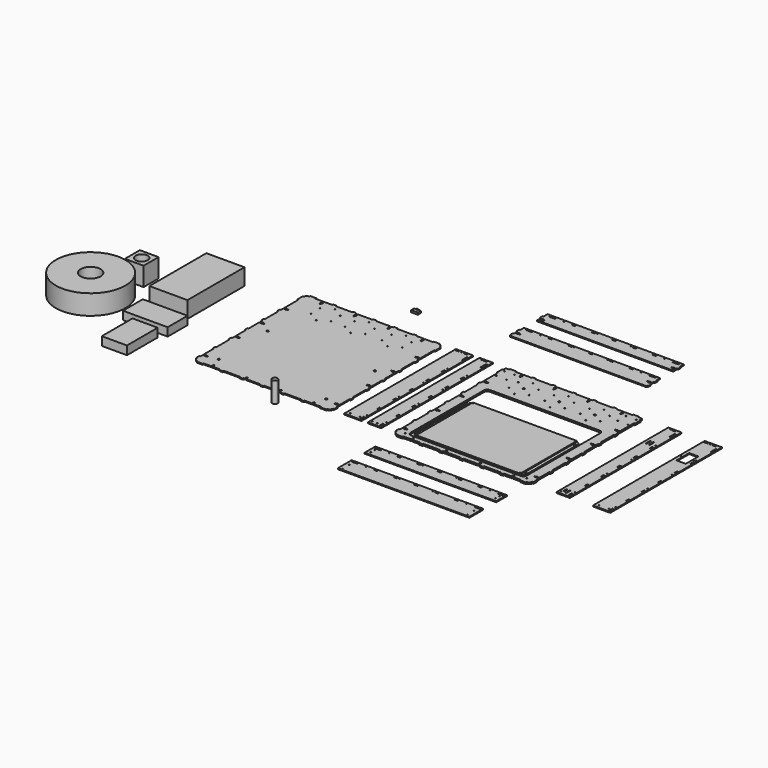
from build123d import *

# Parameters (mm, degrees)
F0_R      = 8
F1_DEPTH  = 62
F2_R      = 1.5
F2_R_2    = 3
F3_DEPTH  = 5
F2_W      = 314
F2_H      = 214
F4_DEPTH  = 2
F2_R_3    = 10
F5_DEPTH  = 3
F2_W_2    = 115
F2_H_2    = 215
F6_DEPTH  = 50
F2_R_4    = 105
F2_R_5    = 30
F7_DEPTH  = 60
F2_W_3    = 135
F2_H_3    = 75
F8_DEPTH  = 25
F2_W_4    = 56.4
F2_H_4    = 56.4
F2_R_6    = 18.5
F9_DEPTH  = 57
F2_W_5    = 76
F2_H_5    = 116
F10_DEPTH = 26
F2_W_6    = 40
F2_H_6    = 408.5
F2_W_7    = 5
F2_H_7    = 13
F2_H_8    = 10
F2_H_9    = 20
F2_H_10   = 12.9999958277
F2_W_8    = 10
F2_H_11   = 3
F11_DEPTH = 3
F2_W_9    = 52
F2_W_10   = 3
F2_W_11   = 28
F2_H_12   = 48
F2_W_12   = 397.0000060797
F2_H_13   = 40
F2_W_13   = 18.5
F2_H_14   = 5
F2_H_15   = 52
F12_DEPTH = 6


# Not quite as in the source:
# - ends of sketch curves that miss each other by under 0.0002 mm in the source are joined
# - a feature names something its author has since deleted; it is built from what else it names


with BuildPart() as f1:
    # F0 (on Top) → F1 (new body)
    with BuildSketch(Plane.XY):
        with Locations((-429.197281599, -257.8284740448)):
            Circle(F0_R)
    extrude(amount=F1_DEPTH)


with BuildPart() as f3:
    # F2 (on Top) → F3 (new body)
    with BuildSketch(Plane.XY):
        with BuildLine():
            Line((102.9999961257, -211.2499983311), (147.2999961257, -211.2499983311))
            Line((147.2999961257, -211.2499983311), (147.2999961257, -208.3499983311))
            Line((147.2999961257, -208.3499983311), (145.7999961257, -208.3499983311))
            Line((145.7999961257, -208.3499983311), (145.7999961257, -205.7499983311))
            Line((145.7999961257, -205.7499983311), (147.2999961257, -205.7499983311))
            Line((147.2999961257, -205.7499983311), (147.2999961257, -202.7499983311))
            Line((147.2999961257, -202.7499983311), (150.6999961257, -202.7499983311))
            Line((150.6999961257, -202.7499983311), (150.6999961257, -205.7499983311))
            Line((150.6999961257, -205.7499983311), (152.1999961257, -205.7499983311))
            Line((152.1999961257, -205.7499983311), (152.1999961257, -208.3499983311))
            Line((152.1999961257, -208.3499983311), (150.6999961257, -208.3499983311))
            Line((150.6999961257, -208.3499983311), (150.6999961257, -211.2499983311))
            Line((150.6999961257, -211.2499983311), (154.9999961257, -211.2499983311))
            Line((154.9999961257, -211.2499983311), (154.9999961257, -214.2499983311))
            Line((154.9999961257, -214.2499983311), (164.9999961257, -214.2499983311))
            Line((164.9999961257, -214.2499983311), (164.9999961257, -211.2499983311))
            Line((164.9999961257, -211.2499983311), (214.9999961257, -211.2499983311))
            Line((214.9999961257, -211.2499983311), (214.9999961257, -214.2499983311))
            Line((214.9999961257, -214.2499983311), (224.9999961257, -214.2499983311))
            Line((224.9999961257, -214.2499983311), (224.9999961257, -211.2499983311))
            Line((224.9999961257, -211.2499983311), (248.2999961257, -211.2499983311))
            Line((248.2999961257, -211.2499983311), (248.2999961257, -208.3499983311))
            Line((248.2999961257, -208.3499983311), (246.7999961257, -208.3499983311))
            Line((246.7999961257, -208.3499983311), (246.7999961257, -205.7499983311))
            Line((246.7999961257, -205.7499983311), (248.2999961257, -205.7499983311))
            Line((248.2999961257, -205.7499983311), (248.2999961257, -202.7499983311))
            Line((248.2999961257, -202.7499983311), (251.6999961257, -202.7499983311))
            Line((251.6999961257, -202.7499983311), (251.6999961257, -205.7499983311))
            Line((251.6999961257, -205.7499983311), (253.1999961257, -205.7499983311))
            Line((253.1999961257, -205.7499983311), (253.1999961257, -208.3499983311))
            Line((253.1999961257, -208.3499983311), (251.6999961257, -208.3499983311))
            Line((251.6999961257, -208.3499983311), (251.6999961257, -211.2499983311))
            Line((251.6999961257, -211.2499983311), (274.9999961257, -211.2499983311))
            Line((274.9999961257, -211.2499983311), (274.9999961257, -214.2499983311))
            Line((274.9999961257, -214.2499983311), (293.4999961257, -214.2499983311))
            Line((293.4999961257, -214.2499983311), (293.4999961257, -211.2499983311))
            ThreePointArc((293.4999961257, -211.2499983311), (300.5710639376, -208.3210661429), (303.4999961257, -201.2499983311))
            Line((303.4999961257, -201.2499983311), (306.4999961257, -201.2499983311))
            Line((306.4999961257, -201.2499983311), (306.4999961257, -188.2500303311))
            Line((306.4999961257, -188.2500303311), (303.4999961257, -188.2500473311))
            Line((303.4999961257, -188.2500473311), (303.4999961257, -179.4499923311))
            Line((303.4999961257, -179.4499923311), (297.0999961257, -179.4499923311))
            Line((297.0999961257, -179.4499923311), (297.0999961257, -180.9499923311))
            Line((297.0999961257, -180.9499923311), (294.4999961257, -180.9499923311))
            Line((294.4999961257, -180.9499923311), (294.4999961257, -179.4499923311))
            Line((294.4999961257, -179.4499923311), (289.4999961257, -179.4499923311))
            Line((289.4999961257, -179.4499923311), (289.4999961257, -176.0499923311))
            Line((289.4999961257, -176.0499923311), (294.4999961257, -176.0499923311))
            Line((294.4999961257, -176.0499923311), (294.4999961257, -174.5499923311))
            Line((294.4999961257, -174.5499923311), (297.0999961257, -174.5499923311))
            Line((297.0999961257, -174.5499923311), (297.0999961257, -176.0499923311))
            Line((297.0999961257, -176.0499923311), (303.4999961257, -176.0499923311))
            Line((303.4999961257, -176.0499923311), (303.4999961257, -138.2500633311))
            Line((303.4999961257, -138.2500633311), (306.4999961257, -138.2500633311))
            Line((306.4999961257, -138.2500633311), (306.4999961257, -128.2500633311))
            Line((306.4999961257, -128.2500633311), (303.4999961257, -128.2500633311))
            Line((303.4999961257, -128.2500633311), (303.4999961257, -78.2500633311))
            Line((303.4999961257, -78.2500633311), (306.4999961257, -78.2500633311))
            Line((306.4999961257, -78.2500633311), (306.4999961257, -68.2500633311))
            Line((306.4999961257, -68.2500633311), (303.4999961257, -68.2500633311))
            Line((303.4999961257, -68.2500633311), (303.4999961257, -58.4499923311))
            Line((303.4999961257, -58.4499923311), (297.0999961257, -58.4499923311))
            Line((297.0999961257, -58.4499923311), (297.0999961257, -59.9499923311))
            Line((297.0999961257, -59.9499923311), (294.4999961257, -59.9499923311))
            Line((294.4999961257, -59.9499923311), (294.4999961257, -58.4499923311))
            Line((294.4999961257, -58.4499923311), (289.4999961257, -58.4499923311))
            Line((289.4999961257, -58.4499923311), (289.4999961257, -55.0499923311))
            Line((289.4999961257, -55.0499923311), (294.4999961257, -55.0499923311))
            Line((294.4999961257, -55.0499923311), (294.4999961257, -53.5499923311))
            Line((294.4999961257, -53.5499923311), (297.0999961257, -53.5499923311))
            Line((297.0999961257, -53.5499923311), (297.0999961257, -55.0499923311))
            Line((297.0999961257, -55.0499923311), (303.4999961257, -55.0499923311))
            Line((303.4999961257, -55.0499923311), (303.4999961257, -16.2500633311))
            Line((303.4999961257, -16.2500633311), (306.4999961257, -16.2500633311))
            Line((306.4999961257, -16.2500633311), (306.4999961257, -6.2500633311))
            Line((306.4999961257, -6.2500633311), (303.4999961257, -6.2500633311))
            Line((303.4999961257, -6.2500633311), (303.4999961257, 33.5500076689))
            Line((303.4999961257, 33.5500076689), (297.0999961257, 33.5500076689))
            Line((297.0999961257, 33.5500076689), (297.0999961257, 32.0500076689))
            Line((297.0999961257, 32.0500076689), (294.4999961257, 32.0500076689))
            Line((294.4999961257, 32.0500076689), (294.4999961257, 33.5500076689))
            Line((294.4999961257, 33.5500076689), (289.4999961257, 33.5500076689))
            Line((289.4999961257, 33.5500076689), (289.4999961257, 36.9500076689))
            Line((289.4999961257, 36.9500076689), (294.4999961257, 36.9500076689))
            Line((294.4999961257, 36.9500076689), (294.4999961257, 38.4500076689))
            Line((294.4999961257, 38.4500076689), (297.0999961257, 38.4500076689))
            Line((297.0999961257, 38.4500076689), (297.0999961257, 36.9500076689))
            Line((297.0999961257, 36.9500076689), (303.4999961257, 36.9500076689))
            Line((303.4999961257, 36.9500076689), (303.4999961257, 45.7499366689))
            Line((303.4999961257, 45.7499366689), (306.4999961257, 45.7499366689))
            Line((306.4999961257, 45.7499366689), (306.4999961257, 55.7499366689))
            Line((306.4999961257, 55.7499366689), (303.4999961257, 55.7499366689))
            Line((303.4999961257, 55.7499366689), (303.4999961257, 105.7499366689))
            Line((303.4999961257, 105.7499366689), (306.4999961257, 105.7499366689))
            Line((306.4999961257, 105.7499366689), (306.4999961257, 115.7499366689))
            Line((306.4999961257, 115.7499366689), (303.4999961257, 115.7499366689))
            Line((303.4999961257, 115.7499366689), (303.4999961257, 124.5500076689))
            Line((303.4999961257, 124.5500076689), (297.0999961257, 124.5500076689))
            Line((297.0999961257, 124.5500076689), (297.0999961257, 123.0500076689))
            Line((297.0999961257, 123.0500076689), (294.4999961257, 123.0500076689))
            Line((294.4999961257, 123.0500076689), (294.4999961257, 124.5500076689))
            Line((294.4999961257, 124.5500076689), (289.4999961257, 124.5500076689))
            Line((289.4999961257, 124.5500076689), (289.4999961257, 127.9500076689))
            Line((289.4999961257, 127.9500076689), (294.4999961257, 127.9500076689))
            Line((294.4999961257, 127.9500076689), (294.4999961257, 129.4500076689))
            Line((294.4999961257, 129.4500076689), (297.0999961257, 129.4500076689))
            Line((297.0999961257, 129.4500076689), (297.0999961257, 127.9500076689))
            Line((297.0999961257, 127.9500076689), (303.4999961257, 127.9500076689))
            Line((303.4999961257, 127.9500076689), (303.4999961257, 181.2500016689))
            Line((303.4999961257, 181.2500016689), (306.4999961257, 181.2500016689))
            Line((306.4999961257, 181.2500016689), (306.4999961257, 201.2500016689))
            Line((306.4999961257, 201.2500016689), (303.4999961257, 201.2500016689))
            Line((303.4999961257, 201.2500016689), (303.4999961257, 211.2500016689))
            Line((303.4999961257, 211.2500016689), (293.4999961257, 211.2500016689))
            Line((293.4999961257, 211.2500016689), (293.4999961257, 214.2500016689))
            Line((293.4999961257, 214.2500016689), (274.9999961257, 214.25))
            Line((274.9999961257, 214.25), (274.9999961257, 211.2500016689))
            Line((274.9999961257, 211.2500016689), (251.6999981257, 211.2500016689))
            Line((251.6999981257, 211.2500016689), (251.6999981257, 204.8500016689))
            Line((251.6999981257, 204.8500016689), (253.1999981257, 204.8500016689))
            Line((253.1999981257, 204.8500016689), (253.1999981257, 202.2500016689))
            Line((253.1999981257, 202.2500016689), (251.6999981257, 202.2500016689))
            Line((251.6999981257, 202.2500016689), (251.6999981257, 197.2500016689))
            Line((251.6999981257, 197.2500016689), (248.2999981257, 197.2500016689))
            Line((248.2999981257, 197.2500016689), (248.2999981257, 202.2500016689))
            Line((248.2999981257, 202.2500016689), (246.7999981257, 202.2500016689))
            Line((246.7999981257, 202.2500016689), (246.7999981257, 204.8500016689))
            Line((246.7999981257, 204.8500016689), (248.2999981257, 204.8500016689))
            Line((248.2999981257, 204.8500016689), (248.2999981257, 211.2500016689))
            Line((248.2999981257, 211.2500016689), (224.9999961257, 211.2500016689))
            Line((224.9999961257, 211.2500016689), (224.9999961257, 214.2500016689))
            Line((224.9999961257, 214.2500016689), (214.9999961257, 214.2500016689))
            Line((214.9999961257, 214.2500016689), (214.9999961257, 211.2500016689))
            Line((214.9999961257, 211.2500016689), (164.9999961257, 211.2500016689))
            Line((164.9999961257, 211.2500016689), (164.9999961257, 214.2500016689))
            Line((164.9999961257, 214.2500016689), (154.9999961257, 214.2500016689))
            Line((154.9999961257, 214.2500016689), (154.9999961257, 211.2500016689))
            Line((154.9999961257, 211.2500016689), (150.6999981257, 211.2500016689))
            Line((150.6999981257, 211.2500016689), (150.6999981257, 204.8500016689))
            Line((150.6999981257, 204.8500016689), (152.1999981257, 204.8500016689))
            Line((152.1999981257, 204.8500016689), (152.1999981257, 202.2500016689))
            Line((152.1999981257, 202.2500016689), (150.6999981257, 202.2500016689))
            Line((150.6999981257, 202.2500016689), (150.6999981257, 197.2500016689))
            Line((150.6999981257, 197.2500016689), (147.2999981257, 197.2500016689))
            Line((147.2999981257, 197.2500016689), (147.2999981257, 202.2500016689))
            Line((147.2999981257, 202.2500016689), (145.7999981257, 202.2500016689))
            Line((145.7999981257, 202.2500016689), (145.7999981257, 204.8500016689))
            Line((145.7999981257, 204.8500016689), (147.2999981257, 204.8500016689))
            Line((147.2999981257, 204.8500016689), (147.2999981257, 211.2500016689))
            Line((147.2999981257, 211.2500016689), (102.9999961257, 211.2500016689))
            Line((102.9999961257, 211.2500016689), (102.9999961257, 214.2500016689))
            Line((102.9999961257, 214.2500016689), (92.9999961257, 214.2500016689))
            Line((92.9999961257, 214.2500016689), (92.9999961257, 211.2500016689))
            Line((92.9999961257, 211.2500016689), (48.6999981257, 211.2500016689))
            Line((48.6999981257, 211.2500016689), (48.6999981257, 204.8500016689))
            Line((48.6999981257, 204.8500016689), (50.1999981257, 204.8500016689))
            Line((50.1999981257, 204.8500016689), (50.1999981257, 202.2500016689))
            Line((50.1999981257, 202.2500016689), (48.6999981257, 202.2500016689))
            Line((48.6999981257, 202.2500016689), (48.6999981257, 197.2500016689))
            Line((48.6999981257, 197.2500016689), (45.2999981257, 197.2500016689))
            Line((45.2999981257, 197.2500016689), (45.2999981257, 202.2500016689))
            Line((45.2999981257, 202.2500016689), (43.7999981257, 202.2500016689))
            Line((43.7999981257, 202.2500016689), (43.7999981257, 204.8500016689))
            Line((43.7999981257, 204.8500016689), (45.2999981257, 204.8500016689))
            Line((45.2999981257, 204.8500016689), (45.2999981257, 211.2500016689))
            Line((45.2999981257, 211.2500016689), (40.9999961257, 211.2500016689))
            Line((40.9999961257, 211.2500016689), (40.9999961257, 214.2500016689))
            Line((40.9999961257, 214.2500016689), (30.9999961257, 214.2500016689))
            Line((30.9999961257, 214.2500016689), (30.9999961257, 211.2500016689))
            Line((30.9999961257, 211.2500016689), (-19.0000038743, 211.2500016689))
            Line((-19.0000038743, 211.2500016689), (-19.0000038743, 214.2500016689))
            Line((-19.0000038743, 214.2500016689), (-29.0000038743, 214.2500016689))
            Line((-29.0000038743, 214.2500016689), (-29.0000038743, 211.2500016689))
            Line((-29.0000038743, 211.2500016689), (-52.3000018743, 211.2500016689))
            Line((-52.3000018743, 211.2500016689), (-52.3000018743, 204.8500016689))
            Line((-52.3000018743, 204.8500016689), (-50.8000018743, 204.8500016689))
            Line((-50.8000018743, 204.8500016689), (-50.8000018743, 202.2500016689))
            Line((-50.8000018743, 202.2500016689), (-52.3000018743, 202.2500016689))
            Line((-52.3000018743, 202.2500016689), (-52.3000018743, 197.2500016689))
            Line((-52.3000018743, 197.2500016689), (-55.7000018743, 197.2500016689))
            Line((-55.7000018743, 197.2500016689), (-55.7000018743, 202.2500016689))
            Line((-55.7000018743, 202.2500016689), (-57.2000018743, 202.2500016689))
            Line((-57.2000018743, 202.2500016689), (-57.2000018743, 204.8500016689))
            Line((-57.2000018743, 204.8500016689), (-55.7000018743, 204.8500016689))
            Line((-55.7000018743, 204.8500016689), (-55.7000018743, 211.2500016689))
            Line((-55.7000018743, 211.2500016689), (-79.0000038743, 211.2500016689))
            Line((-79.0000038743, 211.2500016689), (-79.0000038743, 214.2500016689))
            Line((-79.0000038743, 214.2500016689), (-97.5000038743, 214.2500016689))
            Line((-97.5000038743, 214.2500016689), (-97.5000038743, 211.2500016689))
            Line((-97.5000038743, 211.2500016689), (-107.5000038743, 211.2500016689))
            Line((-107.5000038743, 211.2500016689), (-107.5000038743, 201.2500016689))
            Line((-107.5000038743, 201.2500016689), (-110.5000038743, 201.2500016689))
            Line((-110.5000038743, 201.2500016689), (-110.5000038743, 181.2500016689))
            Line((-110.5000038743, 181.2500016689), (-107.5000038743, 181.2500016689))
            Line((-107.5000038743, 181.2500016689), (-107.5000038743, 127.9500076689))
            Line((-107.5000038743, 127.9500076689), (-101.1000038743, 127.9500076689))
            Line((-101.1000038743, 127.9500076689), (-101.1000038743, 129.4500076689))
            Line((-101.1000038743, 129.4500076689), (-98.5000038743, 129.4500076689))
            Line((-98.5000038743, 129.4500076689), (-98.5000038743, 127.9500076689))
            Line((-98.5000038743, 127.9500076689), (-93.5000038743, 127.9500076689))
            Line((-93.5000038743, 127.9500076689), (-93.5000038743, 124.5500076689))
            Line((-93.5000038743, 124.5500076689), (-98.5000038743, 124.5500076689))
            Line((-98.5000038743, 124.5500076689), (-98.5000038743, 123.0500076689))
            Line((-98.5000038743, 123.0500076689), (-101.1000038743, 123.0500076689))
            Line((-101.1000038743, 123.0500076689), (-101.1000038743, 124.5500076689))
            Line((-101.1000038743, 124.5500076689), (-107.5000038743, 124.5500076689))
            Line((-107.5000038743, 124.5500076689), (-107.5000038743, 115.7499366689))
            Line((-107.5000038743, 115.7499366689), (-110.5000038743, 115.7499366689))
            Line((-110.5000038743, 115.7499366689), (-110.5000038743, 105.7499366689))
            Line((-110.5000038743, 105.7499366689), (-107.5000038743, 105.7499366689))
            Line((-107.5000038743, 105.7499366689), (-107.5000038743, 55.7499366689))
            Line((-107.5000038743, 55.7499366689), (-110.5000038743, 55.7499366689))
            Line((-110.5000038743, 55.7499366689), (-110.5000038743, 45.7499366689))
            Line((-110.5000038743, 45.7499366689), (-107.5000038743, 45.7499366689))
            Line((-107.5000038743, 45.7499366689), (-107.5000038743, 36.9500076689))
            Line((-107.5000038743, 36.9500076689), (-101.1000038743, 36.9500076689))
            Line((-101.1000038743, 36.9500076689), (-101.1000038743, 38.4500076689))
            Line((-101.1000038743, 38.4500076689), (-98.5000038743, 38.4500076689))
            Line((-98.5000038743, 38.4500076689), (-98.5000038743, 36.9500076689))
            Line((-98.5000038743, 36.9500076689), (-93.5000038743, 36.9500076689))
            Line((-93.5000038743, 36.9500076689), (-93.5000038743, 33.5500076689))
            Line((-93.5000038743, 33.5500076689), (-98.5000038743, 33.5500076689))
            Line((-98.5000038743, 33.5500076689), (-98.5000038743, 32.0500076689))
            Line((-98.5000038743, 32.0500076689), (-101.1000038743, 32.0500076689))
            Line((-101.1000038743, 32.0500076689), (-101.1000038743, 33.5500076689))
            Line((-101.1000038743, 33.5500076689), (-107.5000038743, 33.5500076689))
            Line((-107.5000038743, 33.5500076689), (-107.5000038743, -6.2500633311))
            Line((-107.5000038743, -6.2500633311), (-110.5000038743, -6.2500633311))
            Line((-110.5000038743, -6.2500633311), (-110.5000038743, -16.2500633311))
            Line((-110.5000038743, -16.2500633311), (-107.5000038743, -16.2500633311))
            Line((-107.5000038743, -16.2500633311), (-107.5000038743, -55.0499923311))
            Line((-107.5000038743, -55.0499923311), (-101.1000038743, -55.0499923311))
            Line((-101.1000038743, -55.0499923311), (-101.1000038743, -53.5499923311))
            Line((-101.1000038743, -53.5499923311), (-98.5000038743, -53.5499923311))
            Line((-98.5000038743, -53.5499923311), (-98.5000038743, -55.0499923311))
            Line((-98.5000038743, -55.0499923311), (-93.5000038743, -55.0499923311))
            Line((-93.5000038743, -55.0499923311), (-93.5000038743, -58.4499923311))
            Line((-93.5000038743, -58.4499923311), (-98.5000038743, -58.4499923311))
            Line((-98.5000038743, -58.4499923311), (-98.5000038743, -59.9499923311))
            Line((-98.5000038743, -59.9499923311), (-101.1000038743, -59.9499923311))
            Line((-101.1000038743, -59.9499923311), (-101.1000038743, -58.4499923311))
            Line((-101.1000038743, -58.4499923311), (-107.5000038743, -58.4499923311))
            Line((-107.5000038743, -58.4499923311), (-107.5000038743, -68.2500633311))
            Line((-107.5000038743, -68.2500633311), (-110.5000038743, -68.2500633311))
            Line((-110.5000038743, -68.2500633311), (-110.5000038743, -78.2500633311))
            Line((-110.5000038743, -78.2500633311), (-107.5000038743, -78.2500633311))
            Line((-107.5000038743, -78.2500633311), (-107.5000038743, -128.2500633311))
            Line((-107.5000038743, -128.2500633311), (-110.5000038743, -128.2500633311))
            Line((-110.5000038743, -128.2500633311), (-110.5000038743, -138.2500633311))
            Line((-110.5000038743, -138.2500633311), (-107.5000038743, -138.2500633311))
            Line((-107.5000038743, -138.2500633311), (-107.5000038743, -176.0499923311))
            Line((-107.5000038743, -176.0499923311), (-101.1000038743, -176.0499923311))
            Line((-101.1000038743, -176.0499923311), (-101.1000038743, -174.5499923311))
            Line((-101.1000038743, -174.5499923311), (-98.5000038743, -174.5499923311))
            Line((-98.5000038743, -174.5499923311), (-98.5000038743, -176.0499923311))
            Line((-98.5000038743, -176.0499923311), (-93.5000038743, -176.0499923311))
            Line((-93.5000038743, -176.0499923311), (-93.5000038743, -179.4499923311))
            Line((-93.5000038743, -179.4499923311), (-98.5000038743, -179.4499923311))
            Line((-98.5000038743, -179.4499923311), (-98.5000038743, -180.9499923311))
            Line((-98.5000038743, -180.9499923311), (-101.1000038743, -180.9499923311))
            Line((-101.1000038743, -180.9499923311), (-101.1000038743, -179.4499923311))
            Line((-101.1000038743, -179.4499923311), (-107.5000038743, -179.4499923311))
            Line((-107.5000038743, -179.4499923311), (-107.5000038743, -188.2500473311))
            Line((-107.5000038743, -188.2500473311), (-110.5000038743, -188.2500303311))
            Line((-110.5000038743, -188.2500303311), (-110.5000038743, -201.2499983311))
            Line((-110.5000038743, -201.2499983311), (-107.5000038743, -201.2499983311))
            ThreePointArc((-107.5000038743, -201.2499983311), (-104.5710716862, -208.3210661429), (-97.5000038743, -211.2499983311))
            Line((-97.5000038743, -211.2499983311), (-97.5000038743, -214.2499983311))
            Line((-97.5000038743, -214.2499983311), (-79.0000038743, -214.2499983311))
            Line((-79.0000038743, -214.2499983311), (-79.0000038743, -211.2499983311))
            Line((-79.0000038743, -211.2499983311), (-55.7000038743, -211.2499983311))
            Line((-55.7000038743, -211.2499983311), (-55.7000038743, -208.3499983311))
            Line((-55.7000038743, -208.3499983311), (-57.2000038743, -208.3499983311))
            Line((-57.2000038743, -208.3499983311), (-57.2000038743, -205.7499983311))
            Line((-57.2000038743, -205.7499983311), (-55.7000038743, -205.7499983311))
            Line((-55.7000038743, -205.7499983311), (-55.7000038743, -202.7499983311))
            Line((-55.7000038743, -202.7499983311), (-52.3000038743, -202.7499983311))
            Line((-52.3000038743, -202.7499983311), (-52.3000038743, -205.7499983311))
            Line((-52.3000038743, -205.7499983311), (-50.8000038743, -205.7499983311))
            Line((-50.8000038743, -205.7499983311), (-50.8000038743, -208.3499983311))
            Line((-50.8000038743, -208.3499983311), (-52.3000038743, -208.3499983311))
            Line((-52.3000038743, -208.3499983311), (-52.3000038743, -211.2499983311))
            Line((-52.3000038743, -211.2499983311), (-29.0000038743, -211.2499983311))
            Line((-29.0000038743, -211.2499983311), (-29.0000038743, -214.2499983311))
            Line((-29.0000038743, -214.2499983311), (-19.0000038743, -214.2499983311))
            Line((-19.0000038743, -214.2499983311), (-19.0000038743, -211.2499983311))
            Line((-19.0000038743, -211.2499983311), (30.9999961257, -211.2499983311))
            Line((30.9999961257, -211.2499983311), (30.9999961257, -214.2499983311))
            Line((30.9999961257, -214.2499983311), (40.9999961257, -214.2499983311))
            Line((40.9999961257, -214.2499983311), (40.9999961257, -211.2499983311))
            Line((40.9999961257, -211.2499983311), (45.2999961257, -211.2499983311))
            Line((45.2999961257, -211.2499983311), (45.2999961257, -208.3499983311))
            Line((45.2999961257, -208.3499983311), (43.7999961257, -208.3499983311))
            Line((43.7999961257, -208.3499983311), (43.7999961257, -205.7499983311))
            Line((43.7999961257, -205.7499983311), (45.2999961257, -205.7499983311))
            Line((45.2999961257, -205.7499983311), (45.2999961257, -202.7499983311))
            Line((45.2999961257, -202.7499983311), (48.6999961257, -202.7499983311))
            Line((48.6999961257, -202.7499983311), (48.6999961257, -205.7499983311))
            Line((48.6999961257, -205.7499983311), (50.1999961257, -205.7499983311))
            Line((50.1999961257, -205.7499983311), (50.1999961257, -208.3499983311))
            Line((50.1999961257, -208.3499983311), (48.6999961257, -208.3499983311))
            Line((48.6999961257, -208.3499983311), (48.6999961257, -211.2499983311))
            Line((48.6999961257, -211.2499983311), (92.9999961257, -211.2499983311))
            Line((92.9999961257, -211.2499983311), (92.9999961257, -214.2499983311))
            Line((92.9999961257, -214.2499983311), (102.9999961257, -214.2499983311))
            Line((102.9999961257, -214.2499983311), (102.9999961257, -211.2499983311))
        make_face()
        with Locations((-85.5000038743, -196.2499983311)):
            Circle(F2_R, mode=Mode.SUBTRACT)
        with BuildLine():
            ThreePointArc((273.4999961257, -186.2499983311), (270.5710639376, -193.3210661429), (263.4999961257, -196.2499983311))
            Line((263.4999961257, -196.2499983311), (-67.5000038743, -196.2499983311))
            ThreePointArc((-67.5000038743, -196.2499983311), (-74.5710716862, -193.3210661429), (-77.5000038743, -186.2499983311))
            Line((-77.5000038743, -186.2499983311), (-77.5000038743, 91.2500016689))
            ThreePointArc((-77.5000038743, 91.2500016689), (-74.5710716862, 98.3210694808), (-67.5000038743, 101.2500016689))
            Line((-67.5000038743, 101.2500016689), (263.4999961257, 101.2500016689))
            ThreePointArc((263.4999961257, 101.2500016689), (270.5710639376, 98.3210694808), (273.4999961257, 91.2500016689))
            Line((273.4999961257, 91.2500016689), (273.4999961257, -186.2499983311))
        make_face(mode=Mode.SUBTRACT)
        with Locations((281.4999961257, -196.2499983311)):
            Circle(F2_R, mode=Mode.SUBTRACT)
        with Locations((-9.5000038743, 121.2500016689)):
            Circle(F2_R, mode=Mode.SUBTRACT)
        with Locations((-39.8108930068, 138.7500016689)):
            Circle(F2_R, mode=Mode.SUBTRACT)
        with Locations((20.8108852582, 138.7500016689)):
            Circle(F2_R, mode=Mode.SUBTRACT)
        with Locations((97.9999961257, 121.2500016689)):
            Circle(F2_R, mode=Mode.SUBTRACT)
        with Locations((67.6891069932, 138.7500016689)):
            Circle(F2_R, mode=Mode.SUBTRACT)
        with Locations((-101.0000038743, 166.7500016689)):
            Circle(F2_R, mode=Mode.SUBTRACT)
        with Locations((-70.0000038743, 166.7500016689)):
            Circle(F2_R, mode=Mode.SUBTRACT)
        with Locations((-9.5000038743, 156.2500016689)):
            Circle(F2_R_2, mode=Mode.SUBTRACT)
        with Locations((-39.8108930068, 173.7500016689)):
            Circle(F2_R, mode=Mode.SUBTRACT)
        with Locations((-101.0000038743, 197.7500016689)):
            Circle(F2_R, mode=Mode.SUBTRACT)
        with Locations((-70.0000038743, 197.7500016689)):
            Circle(F2_R, mode=Mode.SUBTRACT)
        with Locations((-9.5000038743, 191.2500016689)):
            Circle(F2_R, mode=Mode.SUBTRACT)
        with Locations((20.8108852582, 173.7500016689)):
            Circle(F2_R, mode=Mode.SUBTRACT)
        with Locations((97.9999961257, 156.2500016689)):
            Circle(F2_R_2, mode=Mode.SUBTRACT)
        with Locations((67.6891069932, 173.7500016689)):
            Circle(F2_R, mode=Mode.SUBTRACT)
        with Locations((97.9999961257, 191.2500016689)):
            Circle(F2_R, mode=Mode.SUBTRACT)
        with Locations((128.3108852582, 138.7500016689)):
            Circle(F2_R, mode=Mode.SUBTRACT)
        with Locations((205.4999961257, 121.2500016689)):
            Circle(F2_R, mode=Mode.SUBTRACT)
        with Locations((175.1891069932, 138.7500016689)):
            Circle(F2_R, mode=Mode.SUBTRACT)
        with Locations((235.8108852582, 138.7500016689)):
            Circle(F2_R, mode=Mode.SUBTRACT)
        with Locations((128.3108852582, 173.7500016689)):
            Circle(F2_R, mode=Mode.SUBTRACT)
        with Locations((205.4999961257, 156.2500016689)):
            Circle(F2_R_2, mode=Mode.SUBTRACT)
        with Locations((175.1891069932, 173.7500016689)):
            Circle(F2_R, mode=Mode.SUBTRACT)
        with Locations((205.4999961257, 191.2500016689)):
            Circle(F2_R, mode=Mode.SUBTRACT)
        with Locations((235.8108852582, 173.7500016689)):
            Circle(F2_R, mode=Mode.SUBTRACT)
        with Locations((265.9999961257, 166.7500016689)):
            Circle(F2_R, mode=Mode.SUBTRACT)
        with Locations((296.9999961257, 166.7500016689)):
            Circle(F2_R, mode=Mode.SUBTRACT)
        with Locations((265.9999961257, 197.7500016689)):
            Circle(F2_R, mode=Mode.SUBTRACT)
        with Locations((296.9999961257, 197.7500016689)):
            Circle(F2_R, mode=Mode.SUBTRACT)
    extrude(amount=F3_DEPTH)


with BuildPart() as f3b:
    # F2 (on Top) → F3, piece 2 (new body)
    with BuildSketch(Plane.XY):
        with Locations((97.9999961257, -80.7499983311)):
            Rectangle(F2_W, F2_H)
        with Locations((-56.5000038743, -185.2499983311)):
            Circle(F2_R, mode=Mode.SUBTRACT)
        with Locations((-56.5000038743, 23.7500016689)):
            Circle(F2_R, mode=Mode.SUBTRACT)
        with Locations((252.4999961257, -185.2499983311)):
            Circle(F2_R, mode=Mode.SUBTRACT)
        with Locations((252.4999961257, 23.7500016689)):
            Circle(F2_R, mode=Mode.SUBTRACT)
    extrude(amount=F3_DEPTH)

    # F2 (on Top) → F4 (join)
    with BuildSketch(Plane.XY):
        with BuildLine():
            ThreePointArc((-59.0000038743, 26.2500016689), (-66.0710716862, 23.3210694808), (-69.0000038743, 16.2500016689))
            Line((-69.0000038743, 16.2500016689), (-69.0000038743, -177.7499983311))
            ThreePointArc((-69.0000038743, -177.7499983311), (-66.0710716862, -184.8210661429), (-59.0000038743, -187.7499983311))
            Line((-59.0000038743, -187.7499983311), (-59.0000038743, 26.2500016689))
        make_face()
        with Locations((-64.0000038743, -172.7499983311)):
            Circle(F2_R_2, mode=Mode.SUBTRACT)
        with Locations((-64.0000038743, 11.2500016689)):
            Circle(F2_R_2, mode=Mode.SUBTRACT)
        with BuildLine():
            ThreePointArc((264.9999961257, 16.2500016689), (262.0710639376, 23.3210694808), (254.9999961257, 26.2500016689))
            Line((254.9999961257, 26.2500016689), (254.9999961257, -187.7499983311))
            ThreePointArc((254.9999961257, -187.7499983311), (262.0710639376, -184.8210661429), (264.9999961257, -177.7499983311))
            Line((264.9999961257, -177.7499983311), (264.9999961257, 16.2500016689))
        make_face()
        with Locations((259.9999961257, -172.7499983311)):
            Circle(F2_R_2, mode=Mode.SUBTRACT)
        with Locations((259.9999961257, 11.2500016689)):
            Circle(F2_R_2, mode=Mode.SUBTRACT)
    extrude(amount=F4_DEPTH)


with BuildPart() as f5:
    # F2 (on Top) → F5 (new body)
    with BuildSketch(Plane.XY):
        with BuildLine():
            Line((-499.6031921292, -211.2499983311), (-455.3031921292, -211.2499983311))
            Line((-455.3031921292, -211.2499983311), (-455.3031921292, -208.3499983311))
            Line((-455.3031921292, -208.3499983311), (-456.8031921292, -208.3499983311))
            Line((-456.8031921292, -208.3499983311), (-456.8031921292, -205.7499983311))
            Line((-456.8031921292, -205.7499983311), (-455.3031921292, -205.7499983311))
            Line((-455.3031921292, -205.7499983311), (-455.3031921292, -202.7499983311))
            Line((-455.3031921292, -202.7499983311), (-451.9031921292, -202.7499983311))
            Line((-451.9031921292, -202.7499983311), (-451.9031921292, -205.7499983311))
            Line((-451.9031921292, -205.7499983311), (-450.4031921292, -205.7499983311))
            Line((-450.4031921292, -205.7499983311), (-450.4031921292, -208.3499983311))
            Line((-450.4031921292, -208.3499983311), (-451.9031921292, -208.3499983311))
            Line((-451.9031921292, -208.3499983311), (-451.9031921292, -211.2499983311))
            Line((-451.9031921292, -211.2499983311), (-447.6031921292, -211.2499983311))
            Line((-447.6031921292, -211.2499983311), (-447.6031921292, -214.2499983311))
            Line((-447.6031921292, -214.2499983311), (-437.6031921292, -214.2499983311))
            Line((-437.6031921292, -214.2499983311), (-437.6031921292, -211.2499983311))
            Line((-437.6031921292, -211.2499983311), (-387.6031921292, -211.2499983311))
            Line((-387.6031921292, -211.2499983311), (-387.6031921292, -214.2499983311))
            Line((-387.6031921292, -214.2499983311), (-377.6031921292, -214.2499983311))
            Line((-377.6031921292, -214.2499983311), (-377.6031921292, -211.2499983311))
            Line((-377.6031921292, -211.2499983311), (-354.3031921292, -211.2499983311))
            Line((-354.3031921292, -211.2499983311), (-354.3031921292, -208.3499983311))
            Line((-354.3031921292, -208.3499983311), (-355.8031921292, -208.3499983311))
            Line((-355.8031921292, -208.3499983311), (-355.8031921292, -205.7499983311))
            Line((-355.8031921292, -205.7499983311), (-354.3031921292, -205.7499983311))
            Line((-354.3031921292, -205.7499983311), (-354.3031921292, -202.7499983311))
            Line((-354.3031921292, -202.7499983311), (-350.9031921292, -202.7499983311))
            Line((-350.9031921292, -202.7499983311), (-350.9031921292, -205.7499983311))
            Line((-350.9031921292, -205.7499983311), (-349.4031921292, -205.7499983311))
            Line((-349.4031921292, -205.7499983311), (-349.4031921292, -208.3499983311))
            Line((-349.4031921292, -208.3499983311), (-350.9031921292, -208.3499983311))
            Line((-350.9031921292, -208.3499983311), (-350.9031921292, -211.2499983311))
            Line((-350.9031921292, -211.2499983311), (-327.6031921292, -211.2499983311))
            Line((-327.6031921292, -211.2499983311), (-327.6031921292, -214.2499983311))
            Line((-327.6031921292, -214.2499983311), (-309.1031921292, -214.2499983311))
            Line((-309.1031921292, -214.2499983311), (-309.1031921292, -211.2499983311))
            ThreePointArc((-309.1031921292, -211.2499983311), (-302.0321243174, -208.3210661429), (-299.1031921292, -201.2499983311))
            Line((-299.1031921292, -201.2499983311), (-296.1031921292, -201.2499983311))
            Line((-296.1031921292, -201.2499983311), (-296.1031921292, -188.2500303311))
            Line((-296.1031921292, -188.2500303311), (-299.1031921292, -188.2500473311))
            Line((-299.1031921292, -188.2500473311), (-299.1031921292, -179.4499923311))
            Line((-299.1031921292, -179.4499923311), (-305.5031921292, -179.4499923311))
            Line((-305.5031921292, -179.4499923311), (-305.5031921292, -180.9499923311))
            Line((-305.5031921292, -180.9499923311), (-308.1031921292, -180.9499923311))
            Line((-308.1031921292, -180.9499923311), (-308.1031921292, -179.4499923311))
            Line((-308.1031921292, -179.4499923311), (-313.1031921292, -179.4499923311))
            Line((-313.1031921292, -179.4499923311), (-313.1031921292, -176.0499923311))
            Line((-313.1031921292, -176.0499923311), (-308.1031921292, -176.0499923311))
            Line((-308.1031921292, -176.0499923311), (-308.1031921292, -174.5499923311))
            Line((-308.1031921292, -174.5499923311), (-305.5031921292, -174.5499923311))
            Line((-305.5031921292, -174.5499923311), (-305.5031921292, -176.0499923311))
            Line((-305.5031921292, -176.0499923311), (-299.1031921292, -176.0499923311))
            Line((-299.1031921292, -176.0499923311), (-299.1031921292, -138.2500633311))
            Line((-299.1031921292, -138.2500633311), (-296.1031921292, -138.2500633311))
            Line((-296.1031921292, -138.2500633311), (-296.1031921292, -128.2500633311))
            Line((-296.1031921292, -128.2500633311), (-299.1031921292, -128.2500633311))
            Line((-299.1031921292, -128.2500633311), (-299.1031921292, -78.2500633311))
            Line((-299.1031921292, -78.2500633311), (-296.1031921292, -78.2500633311))
            Line((-296.1031921292, -78.2500633311), (-296.1031921292, -68.2500633311))
            Line((-296.1031921292, -68.2500633311), (-299.1031921292, -68.2500633311))
            Line((-299.1031921292, -68.2500633311), (-299.1031921292, -58.4499923311))
            Line((-299.1031921292, -58.4499923311), (-305.5031921292, -58.4499923311))
            Line((-305.5031921292, -58.4499923311), (-305.5031921292, -59.9499923311))
            Line((-305.5031921292, -59.9499923311), (-308.1031921292, -59.9499923311))
            Line((-308.1031921292, -59.9499923311), (-308.1031921292, -58.4499923311))
            Line((-308.1031921292, -58.4499923311), (-313.1031921292, -58.4499923311))
            Line((-313.1031921292, -58.4499923311), (-313.1031921292, -55.0499923311))
            Line((-313.1031921292, -55.0499923311), (-308.1031921292, -55.0499923311))
            Line((-308.1031921292, -55.0499923311), (-308.1031921292, -53.5499923311))
            Line((-308.1031921292, -53.5499923311), (-305.5031921292, -53.5499923311))
            Line((-305.5031921292, -53.5499923311), (-305.5031921292, -55.0499923311))
            Line((-305.5031921292, -55.0499923311), (-299.1031921292, -55.0499923311))
            Line((-299.1031921292, -55.0499923311), (-299.1031921292, -16.2500633311))
            Line((-299.1031921292, -16.2500633311), (-296.1031921292, -16.2500633311))
            Line((-296.1031921292, -16.2500633311), (-296.1031921292, -6.2500633311))
            Line((-296.1031921292, -6.2500633311), (-299.1031921292, -6.2500633311))
            Line((-299.1031921292, -6.2500633311), (-299.1031921292, 33.5500076689))
            Line((-299.1031921292, 33.5500076689), (-305.5031921292, 33.5500076689))
            Line((-305.5031921292, 33.5500076689), (-305.5031921292, 32.0500076689))
            Line((-305.5031921292, 32.0500076689), (-308.1031921292, 32.0500076689))
            Line((-308.1031921292, 32.0500076689), (-308.1031921292, 33.5500076689))
            Line((-308.1031921292, 33.5500076689), (-313.1031921292, 33.5500076689))
            Line((-313.1031921292, 33.5500076689), (-313.1031921292, 36.9500076689))
            Line((-313.1031921292, 36.9500076689), (-308.1031921292, 36.9500076689))
            Line((-308.1031921292, 36.9500076689), (-308.1031921292, 38.4500076689))
            Line((-308.1031921292, 38.4500076689), (-305.5031921292, 38.4500076689))
            Line((-305.5031921292, 38.4500076689), (-305.5031921292, 36.9500076689))
            Line((-305.5031921292, 36.9500076689), (-299.1031921292, 36.9500076689))
            Line((-299.1031921292, 36.9500076689), (-299.1031921292, 45.7499366689))
            Line((-299.1031921292, 45.7499366689), (-296.1031921292, 45.7499366689))
            Line((-296.1031921292, 45.7499366689), (-296.1031921292, 55.7499366689))
            Line((-296.1031921292, 55.7499366689), (-299.1031921292, 55.7499366689))
            Line((-299.1031921292, 55.7499366689), (-299.1031921292, 105.7499366689))
            Line((-299.1031921292, 105.7499366689), (-296.1031921292, 105.7499366689))
            Line((-296.1031921292, 105.7499366689), (-296.1031921292, 115.7499366689))
            Line((-296.1031921292, 115.7499366689), (-299.1031921292, 115.7499366689))
            Line((-299.1031921292, 115.7499366689), (-299.1031921292, 124.5500076689))
            Line((-299.1031921292, 124.5500076689), (-305.5031921292, 124.5500076689))
            Line((-305.5031921292, 124.5500076689), (-305.5031921292, 123.0500076689))
            Line((-305.5031921292, 123.0500076689), (-308.1031921292, 123.0500076689))
            Line((-308.1031921292, 123.0500076689), (-308.1031921292, 124.5500076689))
            Line((-308.1031921292, 124.5500076689), (-313.1031921292, 124.5500076689))
            Line((-313.1031921292, 124.5500076689), (-313.1031921292, 127.9500076689))
            Line((-313.1031921292, 127.9500076689), (-308.1031921292, 127.9500076689))
            Line((-308.1031921292, 127.9500076689), (-308.1031921292, 129.4500076689))
            Line((-308.1031921292, 129.4500076689), (-305.5031921292, 129.4500076689))
            Line((-305.5031921292, 129.4500076689), (-305.5031921292, 127.9500076689))
            Line((-305.5031921292, 127.9500076689), (-299.1031921292, 127.9500076689))
            Line((-299.1031921292, 127.9500076689), (-299.1031921292, 181.2500016689))
            Line((-299.1031921292, 181.2500016689), (-296.1031921292, 181.2500016689))
            Line((-296.1031921292, 181.2500016689), (-296.1031921292, 201.2500016689))
            Line((-296.1031921292, 201.2500016689), (-299.1031921292, 201.2500016689))
            ThreePointArc((-299.1031921292, 201.2500016689), (-302.0321243174, 208.3210694808), (-309.1031921292, 211.2500016689))
            Line((-309.1031921292, 211.2500016689), (-309.1031921292, 214.2500016689))
            Line((-309.1031921292, 214.2500016689), (-327.6031921292, 214.2500016689))
            Line((-327.6031921292, 214.2500016689), (-327.6031921292, 211.2500016689))
            Line((-327.6031921292, 211.2500016689), (-350.9031901292, 211.2500016689))
            Line((-350.9031901292, 211.2500016689), (-350.9031901292, 204.8500016689))
            Line((-350.9031901292, 204.8500016689), (-349.4031901292, 204.8500016689))
            Line((-349.4031901292, 204.8500016689), (-349.4031901292, 202.2500016689))
            Line((-349.4031901292, 202.2500016689), (-350.9031901292, 202.2500016689))
            Line((-350.9031901292, 202.2500016689), (-350.9031901292, 197.2500016689))
            Line((-350.9031901292, 197.2500016689), (-354.3031901292, 197.2500016689))
            Line((-354.3031901292, 197.2500016689), (-354.3031901292, 202.2500016689))
            Line((-354.3031901292, 202.2500016689), (-355.8031901292, 202.2500016689))
            Line((-355.8031901292, 202.2500016689), (-355.8031901292, 204.8500016689))
            Line((-355.8031901292, 204.8500016689), (-354.3031901292, 204.8500016689))
            Line((-354.3031901292, 204.8500016689), (-354.3031901292, 211.2500016689))
            Line((-354.3031901292, 211.2500016689), (-377.6031921292, 211.2500016689))
            Line((-377.6031921292, 211.2500016689), (-377.6031921292, 214.2500016689))
            Line((-377.6031921292, 214.2500016689), (-387.6031921292, 214.2500016689))
            Line((-387.6031921292, 214.2500016689), (-387.6031921292, 211.2500016689))
            Line((-387.6031921292, 211.2500016689), (-437.6031921292, 211.2500016689))
            Line((-437.6031921292, 211.2500016689), (-437.6031921292, 214.2500016689))
            Line((-437.6031921292, 214.2500016689), (-447.6031921292, 214.2500016689))
            Line((-447.6031921292, 214.2500016689), (-447.6031921292, 211.2500016689))
            Line((-447.6031921292, 211.2500016689), (-451.9031901292, 211.2500016689))
            Line((-451.9031901292, 211.2500016689), (-451.9031901292, 204.8500016689))
            Line((-451.9031901292, 204.8500016689), (-450.4031901292, 204.8500016689))
            Line((-450.4031901292, 204.8500016689), (-450.4031901292, 202.2500016689))
            Line((-450.4031901292, 202.2500016689), (-451.9031901292, 202.2500016689))
            Line((-451.9031901292, 202.2500016689), (-451.9031901292, 197.2500016689))
            Line((-451.9031901292, 197.2500016689), (-455.3031901292, 197.2500016689))
            Line((-455.3031901292, 197.2500016689), (-455.3031901292, 202.2500016689))
            Line((-455.3031901292, 202.2500016689), (-456.8031901292, 202.2500016689))
            Line((-456.8031901292, 202.2500016689), (-456.8031901292, 204.8500016689))
            Line((-456.8031901292, 204.8500016689), (-455.3031901292, 204.8500016689))
            Line((-455.3031901292, 204.8500016689), (-455.3031901292, 211.2500016689))
            Line((-455.3031901292, 211.2500016689), (-499.6031921292, 211.2500016689))
            Line((-499.6031921292, 211.2500016689), (-499.6031921292, 214.2500016689))
            Line((-499.6031921292, 214.2500016689), (-509.6031921292, 214.2500016689))
            Line((-509.6031921292, 214.2500016689), (-509.6031921292, 211.2500016689))
            Line((-509.6031921292, 211.2500016689), (-553.9031901292, 211.2500016689))
            Line((-553.9031901292, 211.2500016689), (-553.9031901292, 204.8500016689))
            Line((-553.9031901292, 204.8500016689), (-552.4031901292, 204.8500016689))
            Line((-552.4031901292, 204.8500016689), (-552.4031901292, 202.2500016689))
            Line((-552.4031901292, 202.2500016689), (-553.9031901292, 202.2500016689))
            Line((-553.9031901292, 202.2500016689), (-553.9031901292, 197.2500016689))
            Line((-553.9031901292, 197.2500016689), (-557.3031901292, 197.2500016689))
            Line((-557.3031901292, 197.2500016689), (-557.3031901292, 202.2500016689))
            Line((-557.3031901292, 202.2500016689), (-558.8031901292, 202.2500016689))
            Line((-558.8031901292, 202.2500016689), (-558.8031901292, 204.8500016689))
            Line((-558.8031901292, 204.8500016689), (-557.3031901292, 204.8500016689))
            Line((-557.3031901292, 204.8500016689), (-557.3031901292, 211.2500016689))
            Line((-557.3031901292, 211.2500016689), (-561.6031921292, 211.2500016689))
            Line((-561.6031921292, 211.2500016689), (-561.6031921292, 214.2500016689))
            Line((-561.6031921292, 214.2500016689), (-571.6031921292, 214.2500016689))
            Line((-571.6031921292, 214.2500016689), (-571.6031921292, 211.2500016689))
            Line((-571.6031921292, 211.2500016689), (-621.6031921292, 211.2500016689))
            Line((-621.6031921292, 211.2500016689), (-621.6031921292, 214.2500016689))
            Line((-621.6031921292, 214.2500016689), (-631.6031921292, 214.2500016689))
            Line((-631.6031921292, 214.2500016689), (-631.6031921292, 211.2500016689))
            Line((-631.6031921292, 211.2500016689), (-654.9031901292, 211.2500016689))
            Line((-654.9031901292, 211.2500016689), (-654.9031901292, 204.8500016689))
            Line((-654.9031901292, 204.8500016689), (-653.4031901292, 204.8500016689))
            Line((-653.4031901292, 204.8500016689), (-653.4031901292, 202.2500016689))
            Line((-653.4031901292, 202.2500016689), (-654.9031901292, 202.2500016689))
            Line((-654.9031901292, 202.2500016689), (-654.9031901292, 197.2500016689))
            Line((-654.9031901292, 197.2500016689), (-658.3031901292, 197.2500016689))
            Line((-658.3031901292, 197.2500016689), (-658.3031901292, 202.2500016689))
            Line((-658.3031901292, 202.2500016689), (-659.8031901292, 202.2500016689))
            Line((-659.8031901292, 202.2500016689), (-659.8031901292, 204.8500016689))
            Line((-659.8031901292, 204.8500016689), (-658.3031901292, 204.8500016689))
            Line((-658.3031901292, 204.8500016689), (-658.3031901292, 211.2500016689))
            Line((-658.3031901292, 211.2500016689), (-681.6031921292, 211.2500016689))
            Line((-681.6031921292, 211.2500016689), (-681.6031921292, 214.2500016689))
            Line((-681.6031921292, 214.2500016689), (-700.1031921292, 214.2500016689))
            Line((-700.1031921292, 214.2500016689), (-700.1031921292, 211.2500016689))
            ThreePointArc((-700.1031921292, 211.2500016689), (-707.1742599411, 208.3210694808), (-710.1031921292, 201.2500016689))
            Line((-710.1031921292, 201.2500016689), (-713.1031921292, 201.2500016689))
            Line((-713.1031921292, 201.2500016689), (-713.1031921292, 181.2500016689))
            Line((-713.1031921292, 181.2500016689), (-710.1031921292, 181.2500016689))
            Line((-710.1031921292, 181.2500016689), (-710.1031921292, 127.9500076689))
            Line((-710.1031921292, 127.9500076689), (-703.7031921292, 127.9500076689))
            Line((-703.7031921292, 127.9500076689), (-703.7031921292, 129.4500076689))
            Line((-703.7031921292, 129.4500076689), (-701.1031921292, 129.4500076689))
            Line((-701.1031921292, 129.4500076689), (-701.1031921292, 127.9500076689))
            Line((-701.1031921292, 127.9500076689), (-696.1031921292, 127.9500076689))
            Line((-696.1031921292, 127.9500076689), (-696.1031921292, 124.5500076689))
            Line((-696.1031921292, 124.5500076689), (-701.1031921292, 124.5500076689))
            Line((-701.1031921292, 124.5500076689), (-701.1031921292, 123.0500076689))
            Line((-701.1031921292, 123.0500076689), (-703.7031921292, 123.0500076689))
            Line((-703.7031921292, 123.0500076689), (-703.7031921292, 124.5500076689))
            Line((-703.7031921292, 124.5500076689), (-710.1031921292, 124.5500076689))
            Line((-710.1031921292, 124.5500076689), (-710.1031921292, 115.7499366689))
            Line((-710.1031921292, 115.7499366689), (-713.1031921292, 115.7499366689))
            Line((-713.1031921292, 115.7499366689), (-713.1031921292, 105.7499366689))
            Line((-713.1031921292, 105.7499366689), (-710.1031921292, 105.7499366689))
            Line((-710.1031921292, 105.7499366689), (-710.1031921292, 55.7499366689))
            Line((-710.1031921292, 55.7499366689), (-713.1031921292, 55.7499366689))
            Line((-713.1031921292, 55.7499366689), (-713.1031921292, 45.7499366689))
            Line((-713.1031921292, 45.7499366689), (-710.1031921292, 45.7499366689))
            Line((-710.1031921292, 45.7499366689), (-710.1031921292, 36.9500076689))
            Line((-710.1031921292, 36.9500076689), (-703.7031921292, 36.9500076689))
            Line((-703.7031921292, 36.9500076689), (-703.7031921292, 38.4500076689))
            Line((-703.7031921292, 38.4500076689), (-701.1031921292, 38.4500076689))
            Line((-701.1031921292, 38.4500076689), (-701.1031921292, 36.9500076689))
            Line((-701.1031921292, 36.9500076689), (-696.1031921292, 36.9500076689))
            Line((-696.1031921292, 36.9500076689), (-696.1031921292, 33.5500076689))
            Line((-696.1031921292, 33.5500076689), (-701.1031921292, 33.5500076689))
            Line((-701.1031921292, 33.5500076689), (-701.1031921292, 32.0500076689))
            Line((-701.1031921292, 32.0500076689), (-703.7031921292, 32.0500076689))
            Line((-703.7031921292, 32.0500076689), (-703.7031921292, 33.5500076689))
            Line((-703.7031921292, 33.5500076689), (-710.1031921292, 33.5500076689))
            Line((-710.1031921292, 33.5500076689), (-710.1031921292, -6.2500633311))
            Line((-710.1031921292, -6.2500633311), (-713.1031921292, -6.2500633311))
            Line((-713.1031921292, -6.2500633311), (-713.1031921292, -16.2500633311))
            Line((-713.1031921292, -16.2500633311), (-710.1031921292, -16.2500633311))
            Line((-710.1031921292, -16.2500633311), (-710.1031921292, -55.0499923311))
            Line((-710.1031921292, -55.0499923311), (-703.7031921292, -55.0499923311))
            Line((-703.7031921292, -55.0499923311), (-703.7031921292, -53.5499923311))
            Line((-703.7031921292, -53.5499923311), (-701.1031921292, -53.5499923311))
            Line((-701.1031921292, -53.5499923311), (-701.1031921292, -55.0499923311))
            Line((-701.1031921292, -55.0499923311), (-696.1031921292, -55.0499923311))
            Line((-696.1031921292, -55.0499923311), (-696.1031921292, -58.4499923311))
            Line((-696.1031921292, -58.4499923311), (-701.1031921292, -58.4499923311))
            Line((-701.1031921292, -58.4499923311), (-701.1031921292, -59.9499923311))
            Line((-701.1031921292, -59.9499923311), (-703.7031921292, -59.9499923311))
            Line((-703.7031921292, -59.9499923311), (-703.7031921292, -58.4499923311))
            Line((-703.7031921292, -58.4499923311), (-710.1031921292, -58.4499923311))
            Line((-710.1031921292, -58.4499923311), (-710.1031921292, -68.2500633311))
            Line((-710.1031921292, -68.2500633311), (-713.1031921292, -68.2500633311))
            Line((-713.1031921292, -68.2500633311), (-713.1031921292, -78.2500633311))
            Line((-713.1031921292, -78.2500633311), (-710.1031921292, -78.2500633311))
            Line((-710.1031921292, -78.2500633311), (-710.1031921292, -128.2500633311))
            Line((-710.1031921292, -128.2500633311), (-713.1031921292, -128.2500633311))
            Line((-713.1031921292, -128.2500633311), (-713.1031921292, -138.2500633311))
            Line((-713.1031921292, -138.2500633311), (-710.1031921292, -138.2500633311))
            Line((-710.1031921292, -138.2500633311), (-710.1031921292, -176.0499923311))
            Line((-710.1031921292, -176.0499923311), (-703.7031921292, -176.0499923311))
            Line((-703.7031921292, -176.0499923311), (-703.7031921292, -174.5499923311))
            Line((-703.7031921292, -174.5499923311), (-701.1031921292, -174.5499923311))
            Line((-701.1031921292, -174.5499923311), (-701.1031921292, -176.0499923311))
            Line((-701.1031921292, -176.0499923311), (-696.1031921292, -176.0499923311))
            Line((-696.1031921292, -176.0499923311), (-696.1031921292, -179.4499923311))
            Line((-696.1031921292, -179.4499923311), (-701.1031921292, -179.4499923311))
            Line((-701.1031921292, -179.4499923311), (-701.1031921292, -180.9499923311))
            Line((-701.1031921292, -180.9499923311), (-703.7031921292, -180.9499923311))
            Line((-703.7031921292, -180.9499923311), (-703.7031921292, -179.4499923311))
            Line((-703.7031921292, -179.4499923311), (-710.1031921292, -179.4499923311))
            Line((-710.1031921292, -179.4499923311), (-710.1031921292, -188.2500473311))
            Line((-710.1031921292, -188.2500473311), (-713.1031921292, -188.2500303311))
            Line((-713.1031921292, -188.2500303311), (-713.1031921292, -201.2499983311))
            Line((-713.1031921292, -201.2499983311), (-710.1031921292, -201.2499983311))
            ThreePointArc((-710.1031921292, -201.2499983311), (-707.1742599411, -208.3210661429), (-700.1031921292, -211.2499983311))
            Line((-700.1031921292, -211.2499983311), (-700.1031921292, -214.2499983311))
            Line((-700.1031921292, -214.2499983311), (-681.6031921292, -214.2499983311))
            Line((-681.6031921292, -214.2499983311), (-681.6031921292, -211.2499983311))
            Line((-681.6031921292, -211.2499983311), (-658.3031921292, -211.2499983311))
            Line((-658.3031921292, -211.2499983311), (-658.3031921292, -208.3499983311))
            Line((-658.3031921292, -208.3499983311), (-659.8031921292, -208.3499983311))
            Line((-659.8031921292, -208.3499983311), (-659.8031921292, -205.7499983311))
            Line((-659.8031921292, -205.7499983311), (-658.3031921292, -205.7499983311))
            Line((-658.3031921292, -205.7499983311), (-658.3031921292, -202.7499983311))
            Line((-658.3031921292, -202.7499983311), (-654.9031921292, -202.7499983311))
            Line((-654.9031921292, -202.7499983311), (-654.9031921292, -205.7499983311))
            Line((-654.9031921292, -205.7499983311), (-653.4031921292, -205.7499983311))
            Line((-653.4031921292, -205.7499983311), (-653.4031921292, -208.3499983311))
            Line((-653.4031921292, -208.3499983311), (-654.9031921292, -208.3499983311))
            Line((-654.9031921292, -208.3499983311), (-654.9031921292, -211.2499983311))
            Line((-654.9031921292, -211.2499983311), (-631.6031921292, -211.2499983311))
            Line((-631.6031921292, -211.2499983311), (-631.6031921292, -214.2499983311))
            Line((-631.6031921292, -214.2499983311), (-621.6031921292, -214.2499983311))
            Line((-621.6031921292, -214.2499983311), (-621.6031921292, -211.2499983311))
            Line((-621.6031921292, -211.2499983311), (-571.6031921292, -211.2499983311))
            Line((-571.6031921292, -211.2499983311), (-571.6031921292, -214.2499983311))
            Line((-571.6031921292, -214.2499983311), (-561.6031921292, -214.2499983311))
            Line((-561.6031921292, -214.2499983311), (-561.6031921292, -211.2499983311))
            Line((-561.6031921292, -211.2499983311), (-557.3031921292, -211.2499983311))
            Line((-557.3031921292, -211.2499983311), (-557.3031921292, -208.3499983311))
            Line((-557.3031921292, -208.3499983311), (-558.8031921292, -208.3499983311))
            Line((-558.8031921292, -208.3499983311), (-558.8031921292, -205.7499983311))
            Line((-558.8031921292, -205.7499983311), (-557.3031921292, -205.7499983311))
            Line((-557.3031921292, -205.7499983311), (-557.3031921292, -202.7499983311))
            Line((-557.3031921292, -202.7499983311), (-553.9031921292, -202.7499983311))
            Line((-553.9031921292, -202.7499983311), (-553.9031921292, -205.7499983311))
            Line((-553.9031921292, -205.7499983311), (-552.4031921292, -205.7499983311))
            Line((-552.4031921292, -205.7499983311), (-552.4031921292, -208.3499983311))
            Line((-552.4031921292, -208.3499983311), (-553.9031921292, -208.3499983311))
            Line((-553.9031921292, -208.3499983311), (-553.9031921292, -211.2499983311))
            Line((-553.9031921292, -211.2499983311), (-509.6031921292, -211.2499983311))
            Line((-509.6031921292, -211.2499983311), (-509.6031921292, -214.2499983311))
            Line((-509.6031921292, -214.2499983311), (-499.6031921292, -214.2499983311))
            Line((-499.6031921292, -214.2499983311), (-499.6031921292, -211.2499983311))
        make_face()
        with Locations((-666.6031921292, -172.7499983311)):
            Circle(F2_R_2, mode=Mode.SUBTRACT)
        with Locations((-342.6031921292, -172.7499983311)):
            Circle(F2_R_2, mode=Mode.SUBTRACT)
        with Locations((-666.6031921292, 11.2500016689)):
            Circle(F2_R_2, mode=Mode.SUBTRACT)
        with Locations((-342.6031921292, 11.2500016689)):
            Circle(F2_R_2, mode=Mode.SUBTRACT)
        with Locations((-612.1031921292, 126.8953830004)):
            Circle(F2_R, mode=Mode.SUBTRACT)
        with Locations((-642.4140812617, 144.3953830004)):
            Circle(F2_R, mode=Mode.SUBTRACT)
        with Locations((-581.7923029968, 144.3953830004)):
            Circle(F2_R, mode=Mode.SUBTRACT)
        with Locations((-508.1031921292, 126.108109951)):
            Circle(F2_R, mode=Mode.SUBTRACT)
        with Locations((-538.4140812617, 143.608109951)):
            Circle(F2_R, mode=Mode.SUBTRACT)
        with Locations((-477.7923029968, 143.608109951)):
            Circle(F2_R, mode=Mode.SUBTRACT)
        with Locations((-397.1031921292, 126.8953830004)):
            Circle(F2_R, mode=Mode.SUBTRACT)
        with Locations((-427.4140812617, 144.3953830004)):
            Circle(F2_R, mode=Mode.SUBTRACT)
        with Locations((-366.7923029968, 144.3953830004)):
            Circle(F2_R, mode=Mode.SUBTRACT)
        with Locations((-612.1031921292, 161.8953830004)):
            Circle(F2_R_3, mode=Mode.SUBTRACT)
        with Locations((-642.4140812617, 179.3953830004)):
            Circle(F2_R, mode=Mode.SUBTRACT)
        with Locations((-612.1031921292, 196.8953830004)):
            Circle(F2_R, mode=Mode.SUBTRACT)
        with Locations((-581.7923029968, 179.3953830004)):
            Circle(F2_R, mode=Mode.SUBTRACT)
        with Locations((-508.1031921292, 161.108109951)):
            Circle(F2_R_3, mode=Mode.SUBTRACT)
        with Locations((-538.4140812617, 178.608109951)):
            Circle(F2_R, mode=Mode.SUBTRACT)
        with Locations((-508.1031921292, 196.108109951)):
            Circle(F2_R, mode=Mode.SUBTRACT)
        with Locations((-477.7923029968, 178.608109951)):
            Circle(F2_R, mode=Mode.SUBTRACT)
        with Locations((-397.1031921292, 161.8953830004)):
            Circle(F2_R_3, mode=Mode.SUBTRACT)
        with Locations((-427.4140812617, 179.3953830004)):
            Circle(F2_R, mode=Mode.SUBTRACT)
        with Locations((-397.1031921292, 196.8953830004)):
            Circle(F2_R, mode=Mode.SUBTRACT)
        with Locations((-366.7923029968, 179.3953830004)):
            Circle(F2_R, mode=Mode.SUBTRACT)
        with Locations((-612.1031921292, 161.8953830004)):
            Circle(F2_R_3)
        with Locations((-508.1031921292, 161.108109951)):
            Circle(F2_R_3)
        with Locations((-397.1031921292, 161.8953830004)):
            Circle(F2_R_3)
    extrude(amount=F5_DEPTH)


with BuildPart() as f6:
    # F2 (on Top) → F6 (new body)
    with BuildSketch(Plane.XY):
        with Locations((-914.2335104942, 53.950006)):
            Rectangle(F2_W_2, F2_H_2)
    extrude(amount=F6_DEPTH)


with BuildPart() as f7:
    # F2 (on Top) → F7 (new body)
    with BuildSketch(Plane.XY):
        with Locations((-1110.3808879852, -101.9591167569)):
            Circle(F2_R_4)
        with Locations((-1110.3808879852, -101.9591167569)):
            Circle(F2_R_5, mode=Mode.SUBTRACT)
    extrude(amount=F7_DEPTH)


with BuildPart() as f8:
    # F2 (on Top) → F8 (new body)
    with BuildSketch(Plane.XY):
        with Locations((-904.2335104942, -115.750065)):
            Rectangle(F2_W_3, F2_H_3)
    extrude(amount=F8_DEPTH)


with BuildPart() as f9:
    # F2 (on Top) → F9 (new body)
    with BuildSketch(Plane.XY):
        with Locations((-1067.1172445297, 36.7578914732)):
            Rectangle(F2_W_4, F2_H_4)
        with Locations((-1067.1172445297, 36.7578914732)):
            Circle(F2_R_6, mode=Mode.SUBTRACT)
    extrude(amount=F9_DEPTH)


with BuildPart() as f10:
    # F2 (on Top) → F10 (new body)
    with BuildSketch(Plane.XY):
        with Locations((-890.3340573311, -229.4109148979)):
            Rectangle(F2_W_5, F2_H_5)
    extrude(amount=F10_DEPTH)


with BuildPart() as f11:
    # F2 (on Top) → F11 (new body)
    with BuildSketch(Plane.XY):
        with Locations((398.3299098015, 5.9605e-06)):
            Rectangle(F2_W_6, F2_H_6)
        with Locations((383.3299098015, -194.2499940395)):
            Circle(F2_R, mode=Mode.SUBTRACT)
        with BuildLine():
            ThreePointArc((398.3299098015, -192.7499940395), (399.3905699733, -193.1893338678), (399.8299098015, -194.2499940395))
            ThreePointArc((399.8299098015, -194.2499940395), (397.2692496297, -195.3106542113), (398.3299098015, -192.7499940395))
        make_face(mode=Mode.SUBTRACT)
        with Locations((412.8299098015, -194.7499940395)):
            Rectangle(F2_W_7, F2_H_7, mode=Mode.SUBTRACT)
        with BuildLine():
            ThreePointArc((390.3299098015, -189.2499940395), (388.8299098015, -190.7499940395), (387.3299098015, -189.2499940395))
            Line((387.3299098015, -189.2499940395), (387.3299098015, -179.2499940395))
            ThreePointArc((387.3299098015, -179.2499940395), (387.7692496297, -178.1893338678), (388.8299098015, -177.7499940395))
            ThreePointArc((388.8299098015, -177.7499940395), (389.8905699733, -178.1893338678), (390.3299098015, -179.2499940395))
            Line((390.3299098015, -179.2499940395), (390.3299098015, -189.2499940395))
        make_face(mode=Mode.SUBTRACT)
        with BuildLine():
            ThreePointArc((399.8299098015, -189.2499940395), (399.3905699733, -190.3106542113), (398.3299098015, -190.7499940395))
            ThreePointArc((398.3299098015, -190.7499940395), (397.2692496297, -190.3106542113), (396.8299098015, -189.2499940395))
            Line((396.8299098015, -189.2499940395), (396.8299098015, -179.2499940395))
            ThreePointArc((396.8299098015, -179.2499940395), (398.3299098015, -177.7499940395), (399.8299098015, -179.2499940395))
            Line((399.8299098015, -179.2499940395), (399.8299098015, -189.2499940395))
        make_face(mode=Mode.SUBTRACT)
        with Locations((412.8299098015, -177.7499940395)):
            Circle(F2_R, mode=Mode.SUBTRACT)
        with Locations((412.8299098015, -133.2499940395)):
            Rectangle(F2_W_7, F2_H_8, mode=Mode.SUBTRACT)
        with Locations((412.8299098015, -73.2499940395)):
            Rectangle(F2_W_7, F2_H_8, mode=Mode.SUBTRACT)
        with Locations((412.8299098015, -56.7499940395)):
            Circle(F2_R, mode=Mode.SUBTRACT)
        with Locations((412.8299098015, -11.2499940395)):
            Rectangle(F2_W_7, F2_H_8, mode=Mode.SUBTRACT)
        with Locations((412.8299098015, 35.2500059605)):
            Circle(F2_R, mode=Mode.SUBTRACT)
        with Locations((412.8299098015, 50.7500059605)):
            Rectangle(F2_W_7, F2_H_8, mode=Mode.SUBTRACT)
        with Locations((412.8299098011, 110.7500059605)):
            Rectangle(F2_W_7, F2_H_8, mode=Mode.SUBTRACT)
        with BuildLine():
            ThreePointArc((390.3299098015, 120.7500059605), (389.8905699733, 119.6893457887), (388.8299098015, 119.2500059605))
            ThreePointArc((388.8299098015, 119.2500059605), (387.7692496297, 119.6893457887), (387.3299098015, 120.7500059605))
            Line((387.3299098015, 120.7500059605), (387.3299098015, 135.7500059605))
            ThreePointArc((387.3299098015, 135.7500059605), (388.8299098015, 137.2500059605), (390.3299098015, 135.7500059605))
            Line((390.3299098015, 135.7500059605), (390.3299098015, 120.7500059605))
        make_face(mode=Mode.SUBTRACT)
        with BuildLine():
            Line((399.8299098015, 135.7500059605), (399.8299098015, 120.7500059605))
            ThreePointArc((399.8299098015, 120.7500059605), (398.3299098015, 119.2500059605), (396.8299098015, 120.7500059605))
            Line((396.8299098015, 120.7500059605), (396.8299098015, 135.7500059605))
            ThreePointArc((396.8299098015, 135.7500059605), (398.3299098015, 137.2500059605), (399.8299098015, 135.7500059605))
        make_face(mode=Mode.SUBTRACT)
        with Locations((412.8299098015, 126.2500059605)):
            Circle(F2_R, mode=Mode.SUBTRACT)
        with Locations((412.8299098015, 191.2500059605)):
            Rectangle(F2_W_7, F2_H_9, mode=Mode.SUBTRACT)
        with Locations((398.3299098015, 210.7500038743)):
            Rectangle(F2_W_6, F2_H_10)
        with Locations((388.3299098015, 212.7500044107)):
            Circle(F2_R, mode=Mode.SUBTRACT)
        with Locations((398.3299098015, 212.7500044107)):
            Rectangle(F2_W_8, F2_H_11, mode=Mode.SUBTRACT)
    extrude(amount=F11_DEPTH)


with BuildPart() as f11b:
    # F2 (on Top) → F11, piece 2 (new body)
    with BuildSketch(Plane.XY):
        with Locations((514.0955723594, 5.9605e-06)):
            Rectangle(F2_W_9, F2_H_6)
        with Locations((498.0955723594, -194.2499940395)):
            Circle(F2_R, mode=Mode.SUBTRACT)
        with Locations((528.0955723594, -194.2499940395)):
            Circle(F2_R, mode=Mode.SUBTRACT)
        with Locations((535.5955723594, -194.7499879599)):
            Rectangle(F2_W_10, F2_H_7, mode=Mode.SUBTRACT)
        with Locations((535.5955723594, -177.7499879599)):
            Circle(F2_R, mode=Mode.SUBTRACT)
        with Locations((535.5955723594, -133.2499879599)):
            Rectangle(F2_W_10, F2_H_8, mode=Mode.SUBTRACT)
        with Locations((535.5955723594, -73.2499879599)):
            Rectangle(F2_W_10, F2_H_8, mode=Mode.SUBTRACT)
        with Locations((535.5955723594, -56.7499879599)):
            Circle(F2_R, mode=Mode.SUBTRACT)
        with Locations((535.5955723594, -11.2499879599)):
            Rectangle(F2_W_10, F2_H_8, mode=Mode.SUBTRACT)
        with Locations((535.5955723594, 35.2500120401)):
            Circle(F2_R, mode=Mode.SUBTRACT)
        with Locations((535.5955723594, 50.7500120401)):
            Rectangle(F2_W_10, F2_H_8, mode=Mode.SUBTRACT)
        with Locations((535.595572359, 110.7500120401)):
            Rectangle(F2_W_10, F2_H_8, mode=Mode.SUBTRACT)
        with Locations((492.0955514908, 122.2500120401)):
            Circle(F2_R, mode=Mode.SUBTRACT)
        with Locations((512.0955514908, 122.2500120401)):
            Rectangle(F2_W_11, F2_H_12, mode=Mode.SUBTRACT)
        with Locations((532.0955514908, 122.2500120401)):
            Circle(F2_R, mode=Mode.SUBTRACT)
        with Locations((535.5955723594, 126.2500120401)):
            Circle(F2_R, mode=Mode.SUBTRACT)
        with Locations((535.5955723594, 191.2500120401)):
            Rectangle(F2_W_10, F2_H_9, mode=Mode.SUBTRACT)
        with Locations((514.0955723594, 210.7500038743)):
            Rectangle(F2_W_9, F2_H_10)
        with Locations((496.0955723594, 212.7500044107)):
            Rectangle(F2_W_8, F2_H_11, mode=Mode.SUBTRACT)
        with Locations((508.5955723594, 212.7500044107)):
            Circle(F2_R, mode=Mode.SUBTRACT)
        with Locations((521.0955723594, 212.7500044107)):
            Rectangle(F2_W_8, F2_H_11, mode=Mode.SUBTRACT)
    extrude(amount=F11_DEPTH)


with BuildPart() as f11c:
    # F2 (on Top) → F11, piece 3 (new body)
    with BuildSketch(Plane.XY):
        with Locations((97.9999991059, -309.9089980079)):
            Rectangle(F2_W_12, F2_H_13)
        with Locations((-90.5000039339, -319.9089980079)):
            Circle(F2_R, mode=Mode.SUBTRACT)
        with Locations((-90.5000039339, -304.9089980079)):
            Circle(F2_R, mode=Mode.SUBTRACT)
        with Locations((-88.2499978542, -295.4089980079)):
            Rectangle(F2_W_13, F2_H_14, mode=Mode.SUBTRACT)
        with Locations((-53.9999978542, -295.4089980079)):
            Circle(F2_R, mode=Mode.SUBTRACT)
        with Locations((-23.9999978542, -295.4089980079)):
            Rectangle(F2_W_8, F2_H_14, mode=Mode.SUBTRACT)
        with Locations((36.0000021458, -295.4089980079)):
            Rectangle(F2_W_8, F2_H_14, mode=Mode.SUBTRACT)
        with Locations((47.0000021458, -295.4089980079)):
            Circle(F2_R, mode=Mode.SUBTRACT)
        with Locations((98.0000021458, -295.4089980079)):
            Rectangle(F2_W_8, F2_H_14, mode=Mode.SUBTRACT)
        with Locations((286.5000021458, -319.9089980079)):
            Circle(F2_R, mode=Mode.SUBTRACT)
        with Locations((149.0000021458, -295.4089980079)):
            Circle(F2_R, mode=Mode.SUBTRACT)
        with Locations((160.0000021458, -295.4089980079)):
            Rectangle(F2_W_8, F2_H_14, mode=Mode.SUBTRACT)
        with Locations((220.0000021458, -295.4089980079)):
            Rectangle(F2_W_8, F2_H_14, mode=Mode.SUBTRACT)
        with Locations((250.0000021458, -295.4089980079)):
            Circle(F2_R, mode=Mode.SUBTRACT)
        with Locations((286.5000021458, -304.9089980079)):
            Circle(F2_R, mode=Mode.SUBTRACT)
        with Locations((284.2500021458, -295.4089980079)):
            Rectangle(F2_W_13, F2_H_14, mode=Mode.SUBTRACT)
    extrude(amount=F11_DEPTH)


with BuildPart() as f11d:
    # F2 (on Top) → F11, piece 4 (new body)
    with BuildSketch(Plane.XY):
        with Locations((97.9999991059, -405.2726975137)):
            Rectangle(F2_W_12, F2_H_15)
        with Locations((-90.5000039339, -426.2726975137)):
            Circle(F2_R, mode=Mode.SUBTRACT)
        with Locations((-90.5000039339, -401.2726975137)):
            Circle(F2_R, mode=Mode.SUBTRACT)
        with Locations((-88.2500039339, -383.7726975138)):
            Rectangle(F2_W_13, F2_H_11, mode=Mode.SUBTRACT)
        with Locations((-54.0000039339, -383.7726975138)):
            Circle(F2_R, mode=Mode.SUBTRACT)
        with Locations((-24.0000039339, -383.7726975138)):
            Rectangle(F2_W_8, F2_H_11, mode=Mode.SUBTRACT)
        with Locations((35.9999960661, -383.7726975138)):
            Rectangle(F2_W_8, F2_H_11, mode=Mode.SUBTRACT)
        with Locations((46.9999960661, -383.7726975138)):
            Circle(F2_R, mode=Mode.SUBTRACT)
        with Locations((97.9999960661, -383.7726975138)):
            Rectangle(F2_W_8, F2_H_11, mode=Mode.SUBTRACT)
        with Locations((148.9999960661, -383.7726975138)):
            Circle(F2_R, mode=Mode.SUBTRACT)
        with Locations((159.9999960661, -383.7726975138)):
            Rectangle(F2_W_8, F2_H_11, mode=Mode.SUBTRACT)
        with Locations((286.5000021458, -426.2726975137)):
            Circle(F2_R, mode=Mode.SUBTRACT)
        with Locations((219.9999960661, -383.7726975138)):
            Rectangle(F2_W_8, F2_H_11, mode=Mode.SUBTRACT)
        with Locations((249.9999960661, -383.7726975138)):
            Circle(F2_R, mode=Mode.SUBTRACT)
        with Locations((286.5000021458, -401.2726975137)):
            Circle(F2_R, mode=Mode.SUBTRACT)
        with Locations((284.2499960661, -383.7726975138)):
            Rectangle(F2_W_13, F2_H_11, mode=Mode.SUBTRACT)
    extrude(amount=F11_DEPTH)


with BuildPart() as f11e:
    # F2 (on Top) → F11, piece 5 (new body)
    with BuildSketch(Plane.XY):
        Polygon((-198.500007391, 451.5279043417), (198.499992609, 451.5279043417), (198.499992609, 458.3278978825), (196.499992609, 458.3278978825), (196.499992609, 459.8278978825), (191.499992609, 459.8278978825), (191.499992609, 463.2278978825), (196.499992609, 463.2278978825), (196.499992609, 464.7278978825), (198.499992609, 464.7278978825), (198.499992609, 491.5279043417), (-198.500007391, 491.5279043417), (-198.500007391, 464.7278978825), (-196.500007391, 464.7278978825), (-196.500007391, 463.2278978825), (-191.500007391, 463.2278978825), (-191.500007391, 459.8278978825), (-196.500007391, 459.8278978825), (-196.500007391, 458.3278978825), (-198.500007391, 458.3278978825), align=None)
        with Locations((-186.250007391, 486.0279043417)):
            Rectangle(F2_W_13, F2_H_14, mode=Mode.SUBTRACT)
        with Locations((-152.000007391, 486.0279043417)):
            Circle(F2_R, mode=Mode.SUBTRACT)
        with Locations((-122.000007391, 486.0279043417)):
            Rectangle(F2_W_8, F2_H_14, mode=Mode.SUBTRACT)
        with Locations((-62.000007391, 486.0279043417)):
            Rectangle(F2_W_8, F2_H_14, mode=Mode.SUBTRACT)
        with Locations((-51.000007391, 486.0279043417)):
            Circle(F2_R, mode=Mode.SUBTRACT)
        with Locations((-7.391e-06, 486.0279043417)):
            Rectangle(F2_W_8, F2_H_14, mode=Mode.SUBTRACT)
        with Locations((50.999992609, 486.0279043417)):
            Circle(F2_R, mode=Mode.SUBTRACT)
        with Locations((61.999992609, 486.0279043417)):
            Rectangle(F2_W_8, F2_H_14, mode=Mode.SUBTRACT)
        with Locations((121.999992609, 486.0279043417)):
            Rectangle(F2_W_8, F2_H_14, mode=Mode.SUBTRACT)
        with Locations((151.999992609, 486.0279043417)):
            Circle(F2_R, mode=Mode.SUBTRACT)
        with Locations((186.249992609, 486.0279043417)):
            Rectangle(F2_W_13, F2_H_14, mode=Mode.SUBTRACT)
        Polygon((198.499992609, 491.5279043417), (198.499992609, 464.7278978825), (199.099992609, 464.7278978825), (199.099992609, 463.2278978825), (205.499992609, 463.2278978825), (205.499992609, 466.5278935432), (205.499992609, 476.5278935432), (205.499992609, 491.5279043417), align=None)
        Polygon((198.499992609, 458.3278978825), (198.499992609, 451.5279043417), (205.499992609, 451.5279043417), (205.499992609, 459.8278978825), (199.099992609, 459.8278978825), (199.099992609, 458.3278978825), align=None)
        with Locations((206.999992609, 471.5278935432)):
            Rectangle(F2_W_10, F2_H_8)
        with Locations((-207.000007391, 471.5278935432)):
            Rectangle(F2_W_10, F2_H_8)
        Polygon((-199.100007391, 464.7278978825), (-198.500007391, 464.7278978825), (-198.500007391, 491.5279043417), (-205.500007391, 491.5279043417), (-205.500007391, 476.5278935432), (-205.500007391, 466.5278935432), (-205.500007391, 463.2278978825), (-199.100007391, 463.2278978825), align=None)
        Polygon((-205.500007391, 451.5279043417), (-198.500007391, 451.5279043417), (-198.500007391, 458.3278978825), (-199.100007391, 458.3278978825), (-199.100007391, 459.8278978825), (-205.500007391, 459.8278978825), align=None)
    extrude(amount=F11_DEPTH)


with BuildPart() as f11f:
    # F2 (on Top) → F11, piece 6 (new body)
    with BuildSketch(Plane.XY):
        Polygon((-198.500007391, 367.4641952515), (-198.500007391, 350.1642048359), (198.4999986887, 350.1642048359), (198.4999986887, 367.4641952515), (196.499992609, 367.4641952515), (196.499992609, 368.9641952515), (191.499992609, 368.9641952515), (191.499992609, 372.3641952515), (196.499992609, 372.3641952515), (196.499992609, 373.8641952515), (198.4999986887, 373.8641952515), (198.4999986887, 402.1642048358), (-198.500007391, 402.1642048358), (-198.500007391, 373.8641952515), (-196.500007391, 373.8641952515), (-196.500007391, 372.3641952515), (-191.500007391, 372.3641952515), (-191.500007391, 368.9641952515), (-196.500007391, 368.9641952515), (-196.500007391, 367.4641952515), align=None)
        with Locations((-186.250007391, 397.6642048358)):
            Rectangle(F2_W_13, F2_H_11, mode=Mode.SUBTRACT)
        with Locations((-152.000007391, 397.6642048358)):
            Circle(F2_R, mode=Mode.SUBTRACT)
        with Locations((-122.000007391, 397.6642048358)):
            Rectangle(F2_W_8, F2_H_11, mode=Mode.SUBTRACT)
        with Locations((-62.000007391, 397.6642048358)):
            Rectangle(F2_W_8, F2_H_11, mode=Mode.SUBTRACT)
        with Locations((-51.000007391, 397.6642048358)):
            Circle(F2_R, mode=Mode.SUBTRACT)
        with Locations((-7.391e-06, 397.6642048358)):
            Rectangle(F2_W_8, F2_H_11, mode=Mode.SUBTRACT)
        with Locations((50.999992609, 397.6642048358)):
            Circle(F2_R, mode=Mode.SUBTRACT)
        with Locations((61.999992609, 397.6642048358)):
            Rectangle(F2_W_8, F2_H_11, mode=Mode.SUBTRACT)
        with Locations((121.999992609, 397.6642048358)):
            Rectangle(F2_W_8, F2_H_11, mode=Mode.SUBTRACT)
        with Locations((151.999992609, 397.6642048358)):
            Circle(F2_R, mode=Mode.SUBTRACT)
        with Locations((186.249992609, 397.6642048358)):
            Rectangle(F2_W_13, F2_H_11, mode=Mode.SUBTRACT)
        Polygon((198.4999986887, 402.1642048358), (198.4999986887, 373.8641952515), (199.099992609, 373.8641952515), (199.099992609, 372.3641952515), (205.499992609, 372.3641952515), (205.4999986887, 378.1642048359), (205.4999986887, 388.1642048359), (205.4999986887, 402.1642048358), align=None)
        with Locations((206.9999986887, 383.1642048359)):
            Rectangle(F2_W_10, F2_H_8)
        with Locations((206.9999986887, 358.1642048359)):
            Rectangle(F2_W_10, F2_H_8)
        Polygon((198.4999986887, 367.4641952515), (198.4999986887, 350.1642048359), (205.4999986887, 350.1642048359), (205.4999986887, 353.1642048359), (205.4999986887, 363.1642048359), (205.4999986887, 368.9641952515), (199.099992609, 368.9641952515), (199.099992609, 367.4641952515), align=None)
        with Locations((-207.000007391, 383.1642048359)):
            Rectangle(F2_W_10, F2_H_8)
        with Locations((-207.000007391, 358.1642048359)):
            Rectangle(F2_W_10, F2_H_8)
        Polygon((-205.500007391, 350.1642048359), (-198.500007391, 350.1642048359), (-198.500007391, 367.4641952515), (-199.100007391, 367.4641952515), (-199.100007391, 368.9641952515), (-205.500007391, 368.9641952515), (-205.500007391, 363.1642048359), (-205.500007391, 353.1642048359), align=None)
        Polygon((-199.100007391, 373.8641952515), (-198.500007391, 373.8641952515), (-198.500007391, 402.1642048358), (-205.500007391, 402.1642048358), (-205.500007391, 388.1642048359), (-205.500007391, 378.1642048359), (-205.500007391, 372.3641952515), (-199.100007391, 372.3641952515), align=None)
    extrude(amount=F11_DEPTH)


with BuildPart() as f11g:
    # F2 (on Top) → F11, piece 7 (new body)
    with BuildSketch(Plane.XY):
        with Locations((-171.500007391, 7.0333e-06)):
            Rectangle(F2_W_6, F2_H_6)
        with Locations((-186.500007391, -194.2499929667)):
            Circle(F2_R, mode=Mode.SUBTRACT)
        with Locations((-171.500007391, -194.2499929667)):
            Circle(F2_R, mode=Mode.SUBTRACT)
        with Locations((-157.000007391, -194.7499929667)):
            Rectangle(F2_W_7, F2_H_7, mode=Mode.SUBTRACT)
        with Locations((-157.000007391, -177.7499929667)):
            Circle(F2_R, mode=Mode.SUBTRACT)
        with Locations((-157.000007391, -133.2499929667)):
            Rectangle(F2_W_7, F2_H_8, mode=Mode.SUBTRACT)
        with Locations((-157.000007391, -73.2499929667)):
            Rectangle(F2_W_7, F2_H_8, mode=Mode.SUBTRACT)
        with Locations((-157.000007391, -56.7499929667)):
            Circle(F2_R, mode=Mode.SUBTRACT)
        with Locations((-157.000007391, -11.2499929667)):
            Rectangle(F2_W_7, F2_H_8, mode=Mode.SUBTRACT)
        with Locations((-157.000007391, 35.2500070333)):
            Circle(F2_R, mode=Mode.SUBTRACT)
        with Locations((-157.000007391, 50.7500070333)):
            Rectangle(F2_W_7, F2_H_8, mode=Mode.SUBTRACT)
        with Locations((-157.0000073914, 110.7500070333)):
            Rectangle(F2_W_7, F2_H_8, mode=Mode.SUBTRACT)
        with Locations((-157.000007391, 126.2500070333)):
            Circle(F2_R, mode=Mode.SUBTRACT)
        with Locations((-157.000007391, 191.2500070333)):
            Rectangle(F2_W_7, F2_H_9, mode=Mode.SUBTRACT)
        with Locations((-171.500007391, 210.7500049472)):
            Rectangle(F2_W_6, F2_H_10)
        with Locations((-181.500007391, 212.7500054836)):
            Circle(F2_R, mode=Mode.SUBTRACT)
        with Locations((-171.500007391, 212.7500054836)):
            Rectangle(F2_W_8, F2_H_11, mode=Mode.SUBTRACT)
    extrude(amount=F11_DEPTH)


with BuildPart() as f11h:
    # F2 (on Top) → F11, piece 8 (new body)
    with BuildSketch(Plane.XY):
        with Locations((-236.8936419189, 7.0333e-06)):
            Rectangle(F2_W_9, F2_H_6)
        with Locations((-252.8936419189, -194.2499929667)):
            Circle(F2_R, mode=Mode.SUBTRACT)
        with Locations((-222.8936419189, -194.2499929667)):
            Circle(F2_R, mode=Mode.SUBTRACT)
        with Locations((-215.3936419189, -194.749986887)):
            Rectangle(F2_W_10, F2_H_7, mode=Mode.SUBTRACT)
        with Locations((-215.3936419189, -177.749986887)):
            Circle(F2_R, mode=Mode.SUBTRACT)
        with Locations((-215.3936419189, -133.249986887)):
            Rectangle(F2_W_10, F2_H_8, mode=Mode.SUBTRACT)
        with Locations((-215.3936419189, -73.249986887)):
            Rectangle(F2_W_10, F2_H_8, mode=Mode.SUBTRACT)
        with Locations((-215.3936419189, -56.749986887)):
            Circle(F2_R, mode=Mode.SUBTRACT)
        with Locations((-215.3936419189, -11.249986887)):
            Rectangle(F2_W_10, F2_H_8, mode=Mode.SUBTRACT)
        with Locations((-215.3936419189, 35.250013113)):
            Circle(F2_R, mode=Mode.SUBTRACT)
        with Locations((-215.3936419189, 50.750013113)):
            Rectangle(F2_W_10, F2_H_8, mode=Mode.SUBTRACT)
        with Locations((-215.3936419193, 110.750013113)):
            Rectangle(F2_W_10, F2_H_8, mode=Mode.SUBTRACT)
        with Locations((-215.3936419189, 126.250013113)):
            Circle(F2_R, mode=Mode.SUBTRACT)
        with Locations((-215.3936419189, 191.250013113)):
            Rectangle(F2_W_10, F2_H_9, mode=Mode.SUBTRACT)
        with Locations((-236.8936419189, 210.7500049472)):
            Rectangle(F2_W_9, F2_H_10)
        with Locations((-254.8936419189, 212.7500054836)):
            Rectangle(F2_W_8, F2_H_11, mode=Mode.SUBTRACT)
        with Locations((-242.3936419189, 212.7500054836)):
            Circle(F2_R, mode=Mode.SUBTRACT)
        with Locations((-229.8936419189, 212.7500054836)):
            Rectangle(F2_W_8, F2_H_11, mode=Mode.SUBTRACT)
    extrude(amount=F11_DEPTH)


with BuildPart() as f12:
    # F2 (on Top) → F12 (new body)
    with BuildSketch(Plane.XY):
        Polygon((-465.8188569283, 313.1877682719), (-465.8188569283, 302.1877682719), (-445.8188569283, 302.1877682719), (-445.8188569283, 313.1877682719), (-449.8188569283, 313.1877682719), align=None)
        with Locations((-460.6212079525, 303.7134706974)):
            Circle(F2_R, mode=Mode.SUBTRACT)
        with Locations((-451.1212079525, 303.7134706974)):
            Circle(F2_R, mode=Mode.SUBTRACT)
        Polygon((-449.8188569283, 313.1877682719), (-445.8188569283, 313.1877682719), (-463.1626069283, 318.0038180991), align=None)
    extrude(amount=F12_DEPTH)


solid = Compound([f1.part, f3.part, f3b.part, f5.part, f6.part, f7.part, f8.part, f9.part, f10.part, f11.part, f11b.part, f11c.part, f11d.part, f11e.part, f11f.part, f11g.part, f11h.part, f12.part])
